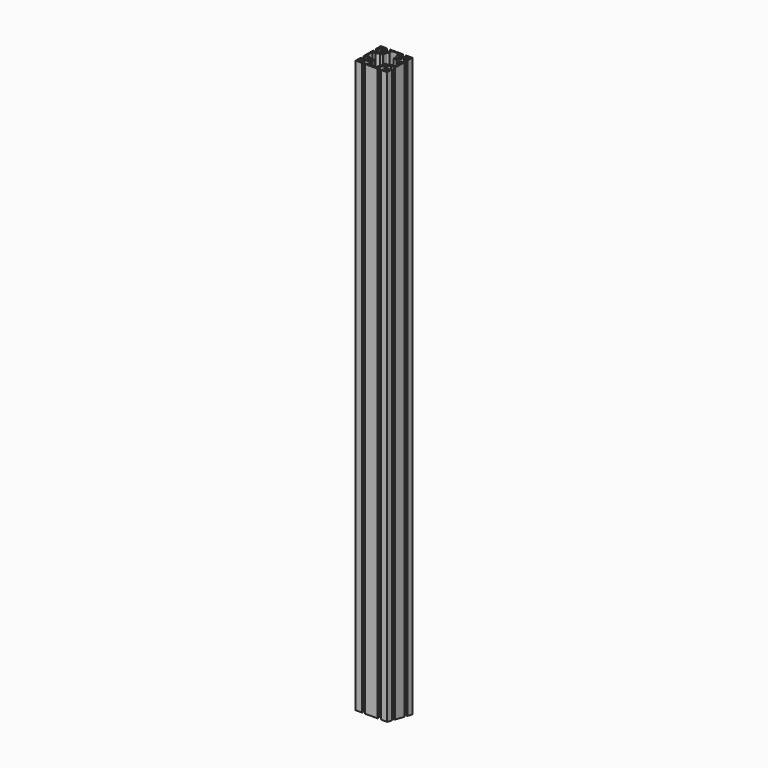
from build123d import *

# Parameters (mm, degrees)
F0_R          = 3
F0_R_2        = 2.5
F1_DEPTH      = 1100.6
F2_R          = 2
F3_R          = 7
F5_DEPTH      = 30
F5_DEPTH_BACK = 30


# Not quite as in the source:
# - a feature names something its author has since deleted; it is built from what else it names


with BuildPart() as f1:
    # F0 (on Top) → F1 (new body)
    with BuildSketch(Plane.XY):
        with BuildLine():
            Line((18.15, -30), (30, -30))
            Line((30, -30), (30, -18.15))
            Line((30, -18.15), (27.5, -18.15))
            Line((27.5, -18.15), (27.5, -20.15))
            Line((27.5, -20.15), (21.5477069044, -20.15))
            ThreePointArc((21.5477069044, -20.15), (19.5, -15), (21.5477069044, -9.85))
            Line((21.5477069044, -9.85), (27.5, -9.85))
            Line((27.5, -9.85), (27.5, -11.85))
            Line((27.5, -11.85), (30, -11.85))
            Line((30, -11.85), (30, 11.85))
            Line((30, 11.85), (27.5, 11.85))
            Line((27.5, 11.85), (27.5, 9.85))
            Line((27.5, 9.85), (21.5477069044, 9.85))
            ThreePointArc((21.5477069044, 9.85), (19.5, 15), (21.5477069044, 20.15))
            Line((21.5477069044, 20.15), (27.5, 20.15))
            Line((27.5, 20.15), (27.5, 18.15))
            Line((27.5, 18.15), (30, 18.15))
            Line((30, 18.15), (30, 30))
            Line((30, 30), (18.15, 30))
            Line((18.15, 30), (18.15, 27.5))
            Line((18.15, 27.5), (20.15, 27.5))
            Line((20.15, 27.5), (20.15, 21.5477069044))
            ThreePointArc((20.15, 21.5477069044), (15, 19.5), (9.85, 21.5477069044))
            Line((9.85, 21.5477069044), (9.85, 27.5))
            Line((9.85, 27.5), (11.85, 27.5))
            Line((11.85, 27.5), (11.85, 30))
            Line((11.85, 30), (-11.85, 30))
            Line((-11.85, 30), (-11.85, 27.5))
            Line((-11.85, 27.5), (-9.85, 27.5))
            Line((-9.85, 27.5), (-9.85, 21.5477069044))
            ThreePointArc((-9.85, 21.5477069044), (-15, 19.5), (-20.15, 21.5477069044))
            Line((-20.15, 21.5477069044), (-20.15, 27.5))
            Line((-20.15, 27.5), (-18.15, 27.5))
            Line((-18.15, 27.5), (-18.15, 30))
            Line((-18.15, 30), (-30, 30))
            Line((-30, 30), (-30, 18.15))
            Line((-30, 18.15), (-27.5, 18.15))
            Line((-27.5, 18.15), (-27.5, 20.15))
            Line((-27.5, 20.15), (-21.5477069044, 20.15))
            ThreePointArc((-21.5477069044, 20.15), (-19.5, 15), (-21.5477069044, 9.85))
            Line((-21.5477069044, 9.85), (-27.5, 9.85))
            Line((-27.5, 9.85), (-27.5, 11.85))
            Line((-27.5, 11.85), (-30, 11.85))
            Line((-30, 11.85), (-30, -11.85))
            Line((-30, -11.85), (-27.5, -11.85))
            Line((-27.5, -11.85), (-27.5, -9.85))
            Line((-27.5, -9.85), (-21.5477069044, -9.85))
            ThreePointArc((-21.5477069044, -9.85), (-19.5, -15), (-21.5477069044, -20.15))
            Line((-21.5477069044, -20.15), (-27.5, -20.15))
            Line((-27.5, -20.15), (-27.5, -18.15))
            Line((-27.5, -18.15), (-30, -18.15))
            Line((-30, -18.15), (-30, -30))
            Line((-30, -30), (-18.15, -30))
            Line((-18.15, -30), (-18.15, -27.5))
            Line((-18.15, -27.5), (-20.15, -27.5))
            Line((-20.15, -27.5), (-20.15, -21.5477069044))
            ThreePointArc((-20.15, -21.5477069044), (-15, -19.5), (-9.85, -21.5477069044))
            Line((-9.85, -21.5477069044), (-9.85, -27.5))
            Line((-9.85, -27.5), (-11.85, -27.5))
            Line((-11.85, -27.5), (-11.85, -30))
            Line((-11.85, -30), (11.85, -30))
            Line((11.85, -30), (11.85, -27.5))
            Line((11.85, -27.5), (9.85, -27.5))
            Line((9.85, -27.5), (9.85, -21.5477069044))
            ThreePointArc((9.85, -21.5477069044), (15, -19.5), (20.15, -21.5477069044))
            Line((20.15, -21.5477069044), (20.15, -27.5))
            Line((20.15, -27.5), (18.15, -27.5))
            Line((18.15, -27.5), (18.15, -30))
        make_face()
        with Locations((-25, -25)):
            Circle(F0_R, mode=Mode.SUBTRACT)
        with Locations((-15, -15)):
            Circle(F0_R_2, mode=Mode.SUBTRACT)
        with Locations((25, -25)):
            Circle(F0_R, mode=Mode.SUBTRACT)
        with Locations((15, -15)):
            Circle(F0_R_2, mode=Mode.SUBTRACT)
        with Locations((-25, 25)):
            Circle(F0_R, mode=Mode.SUBTRACT)
        with Locations((-15, 15)):
            Circle(F0_R_2, mode=Mode.SUBTRACT)
        Polygon((-7, 22), (-7, 27.5), (0, 27.5), (7, 27.5), (7, 22), (10, 16), (10, 10), (16, 10), (22, 7), (27.5, 7), (27.5, 0), (27.5, -7), (22, -7), (16, -10), (10, -10), (10, -16), (7, -22), (7, -27.5), (0, -27.5), (-7, -27.5), (-7, -22), (-10, -16), (-10, -10), (-16, -10), (-22, -7), (-27.5, -7), (-27.5, 0), (-27.5, 7), (-22, 7), (-16, 10), (-10, 10), (-10, 16), align=None, mode=Mode.SUBTRACT)
        with Locations((15, 15)):
            Circle(F0_R_2, mode=Mode.SUBTRACT)
        with Locations((25, 25)):
            Circle(F0_R, mode=Mode.SUBTRACT)
    extrude(amount=F1_DEPTH)

    # F2
    f2_edges = [f1.edges().sort_by_distance(p)[0] for p in [
        (-7, 27.5, 550.3),
        (7, 27.5, 550.3),
    ]]
    fillet(f2_edges, radius=F2_R)

    # F3
    f3_edges = [f1.edges().sort_by_distance(p)[0] for p in [
        (-10, 16, 550.3),
        (10, 16, 550.3),
    ]]
    fillet(f3_edges, radius=F3_R)

    # F4 (on Right) → F5 (cut, two sides)
    with BuildSketch(Plane.YZ) as f5_sk:
        Polygon((-164.2855995683, 38.6458085579), (-188.5911429791, -83.5464097089), (5.6944565892, -122.1922182668), (30, 0), align=None)
    extrude(amount=F5_DEPTH, mode=Mode.SUBTRACT)
    extrude(f5_sk.sketch, amount=-F5_DEPTH_BACK, mode=Mode.SUBTRACT)


solid = f1.part
